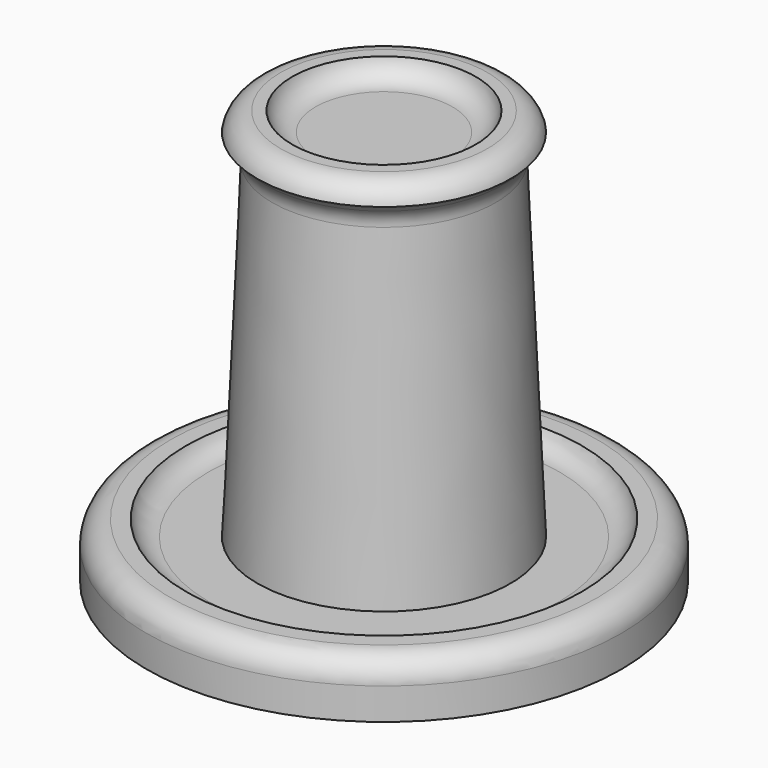
from build123d import *


# Not quite as in the source:
# - a fillet or chamfer that OpenCascade refuses, or shapes differently, is made with other operations: its cross-section is extruded or revolved along the edge and cut away or added


with BuildPart() as f1:
    # F0 (on Front) → F1 (revolve)
    with BuildSketch(Plane.XZ):
        Polygon((-30, 7), (-30, 0), (0, 0), (0, 50), (-11.6, 50), (-11.6, 52.4), (-16, 52.4), (-16, 50), (-14.085106383, 48.085106383), (-16, 5), (-25, 5), (-25, 7), align=None)
    revolve(axis=Axis((0, 0, 15.8572417056), (0, 0, 1)))

    # F2: fillet of radius 3 on 5 edges, made by hand

    # F2_s1 → F2_t2 (revolve)
    with BuildSketch(Plane.XZ):
        with BuildLine():
            ThreePointArc((-22.1715728753, 5), (-23.9036236828, 5.5505102572), (-25, 7))
            Line((-25, 7), (-25, 5))
            Line((-25, 5), (-22.1715728753, 5))
        make_face()
    revolve(axis=Axis((0, 0, 5), (0, 0, 1)))

    # F2_s3 → F2_t4 (revolve)
    with BuildSketch(Plane.XZ):
        with BuildLine():
            ThreePointArc((-14.1437787706, 46.764977662), (-14.3443716648, 47.9844003118), (-15.0194998464, 49.0194998464))
            Line((-15.0194998464, 49.0194998464), (-14.085106383, 48.085106383))
            Line((-14.085106383, 48.085106383), (-14.1437787706, 46.764977662))
        make_face()
    revolve(axis=Axis((0, 0, 48.085106383), (0, 0, 1)))

    # F2_s5 → F2_t6 (revolve)
    with BuildSketch(Plane.XZ):
        with BuildLine():
            ThreePointArc((-8.6606123087, 50), (-10.5579789048, 50.6762099923), (-11.6, 52.4))
            Line((-11.6, 52.4), (-11.6, 50))
            Line((-11.6, 50), (-8.6606123087, 50))
        make_face()
    revolve(axis=Axis((0, 0, 50), (0, 0, 1)))

    # F2_s7 → F2_t8 (revolve, cut)
    with BuildSketch(Plane.XZ):
        with BuildLine():
            ThreePointArc((-27, 7), (-29.1213203436, 6.1213203436), (-30, 4))
            Line((-30, 4), (-30, 7))
            Line((-30, 7), (-27, 7))
        make_face()
    revolve(axis=Axis((0, 0, 7), (0, 0, 1)), mode=Mode.SUBTRACT)

    # F2_s9 → F2_t10 (revolve, cut)
    with BuildSketch(Plane.XZ):
        with BuildLine():
            ThreePointArc((-16, 50), (-14.9579789048, 51.7237900077), (-13.0606123087, 52.4))
            Line((-13.0606123087, 52.4), (-16, 52.4))
            Line((-16, 52.4), (-16, 50))
        make_face()
    revolve(axis=Axis((0, 0, 52.4), (0, 0, 1)), mode=Mode.SUBTRACT)


solid = f1.part
